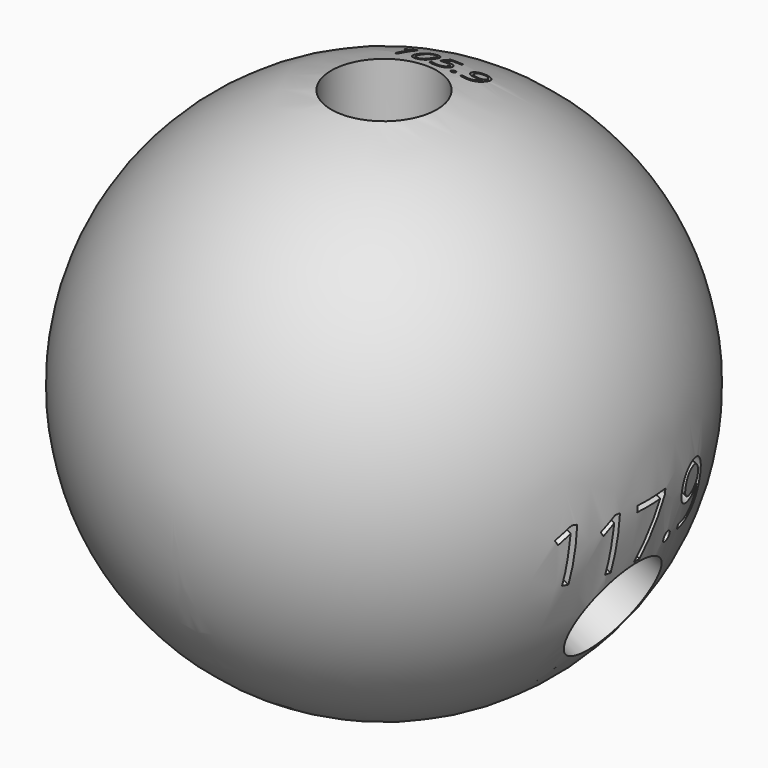
from build123d import *

# Parameters (mm, degrees)
F4_R          = 3.175
F5_DEPTH      = 25.4
F7_TEXT_SIZE  = 2.1726426591
F8_DEPTH      = 10.16
F10_ANGLE     = 117.9
F12_TEXT_SIZE = 4.4907268602
F13_DEPTH     = 10.16
F15_ANGLE     = -136.2
F17_TEXT_SIZE = 1.5241931477
F18_DEPTH     = 10.16


# Not quite as in the source:
# - Text() gives the source's letters only with a copy of the font that has no kerning and outlines rounded to 1/6400 em; it was checked with that copy


with BuildPart() as f2:
    # F0 (on Right) → F2 (revolve)
    with BuildSketch(Plane.YZ):
        with BuildLine():
            Line((15.875, 0), (-15.875, 0))
            ThreePointArc((-15.875, 0), (0, -15.875), (15.875, 0))
        make_face()
    revolve(axis=Axis((0, 0, 0), (0, -1, 0)))

    # F7 (on offset) → F8 (cut)
    with BuildSketch(Plane.XY.offset(19.05)):
        with Locations((-2.875527367, 3.6710030399)):
            Text('105.9', F7_TEXT_SIZE, font='Open Sans', text_align=(TextAlign.LEFT, TextAlign.BOTTOM))
    extrude(amount=-F8_DEPTH, mode=Mode.SUBTRACT)

    # F12 (on offset) → F13 (cut)
    with BuildSketch(Plane(origin=(16.8357352532, 0, -8.9140629617), x_dir=(0, 1, 0), z_dir=(0.8837656301, 0, -0.4679298143))):
        with Locations((-6.0638728319, 3.3226958476)):
            Text('117.9', F12_TEXT_SIZE, font='Open Sans', text_align=(TextAlign.LEFT, TextAlign.BOTTOM))
    extrude(amount=-F13_DEPTH, mode=Mode.SUBTRACT)

    # F17 (on offset) → F18 (cut)
    with BuildSketch(Plane(origin=(-13.1853274622, 0, -13.7495323453), x_dir=(0.7217602281, 0, -0.6921431739), z_dir=(-0.6921431739, 0, -0.7217602281))):
        with Locations((-2.0607443439, 3.7946992088)):
            Text('136.2', F17_TEXT_SIZE, font='Open Sans', text_align=(TextAlign.LEFT, TextAlign.BOTTOM))
    extrude(amount=-F18_DEPTH, mode=Mode.SUBTRACT)


with BuildPart() as f5:
    # F4 (on offset) → F5 (new body)
    with BuildSketch(Plane.XY.offset(6.35)):
        Circle(F4_R)
    extrude(amount=F5_DEPTH)


with BuildPart() as f10_1:
    # F10: copy of F5
    add(f5.part.rotate(Axis((0, -1.2904852629, 0), (0, 1, 0)), F10_ANGLE))


with BuildPart() as f15_1:
    # F15: copy of F5
    add(f5.part.rotate(Axis((0, -1.8435455859, 0), (0, 1, 0)), F15_ANGLE))


with BuildPart() as f2_1:
    add(f2.part)

    # F19: cut F5, F15_1, F10_1
    add(f5.part, mode=Mode.SUBTRACT)
    add(f15_1.part, mode=Mode.SUBTRACT)
    add(f10_1.part, mode=Mode.SUBTRACT)


solid = f2_1.part
